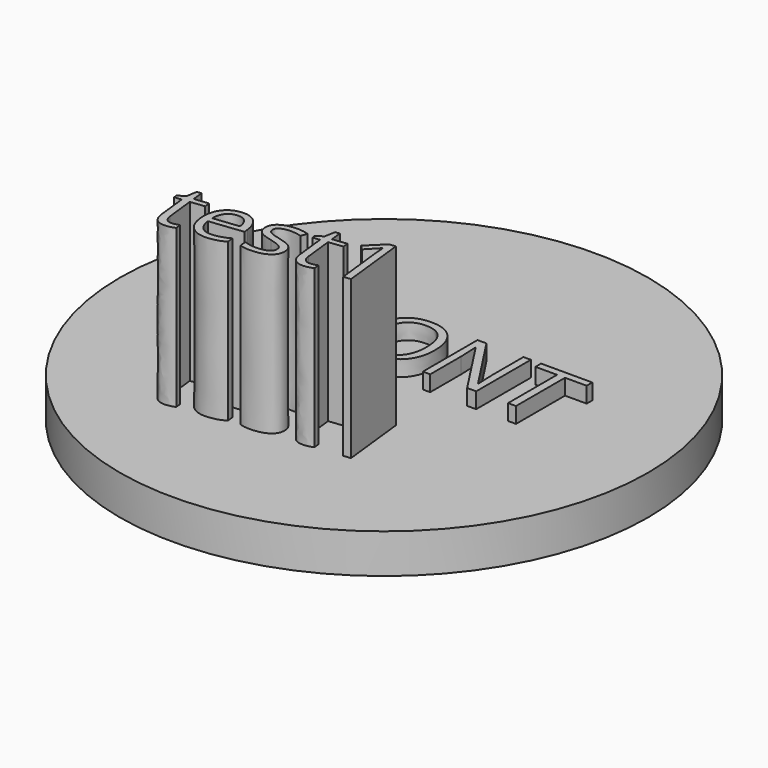
from build123d import *

# Parameters (mm, degrees)
F0_R         = 42.5666121287
F1_DEPTH     = 6.35
F2_TEXT_SIZE = 15.4234249041
F3_DEPTH     = 2.54
F4_TEXT_SIZE = 13.8114629937
F5_DEPTH     = 2.54
F6_TEXT_SIZE = 13.8114629937
F7_DEPTH     = 8.89
F8_TEXT_SIZE = 14.7895900429
F9_DEPTH     = 25.4


# Not quite as in the source:
# - Text() gives the source's letters only with a copy of the font that has no kerning and outlines rounded to 1/6400 em; it was checked with that copy


with BuildPart() as f1:
    # F0 (on Top) → F1 (new body)
    with BuildSketch(Plane.XY):
        Circle(F0_R)
    extrude(amount=F1_DEPTH)

    # F2 (on face) → F3 (join)
    with BuildSketch(Plane.XY.offset(6.35)):
        with Locations((-24.7606217465, 0)):
            Text('FRONT', F2_TEXT_SIZE, font='Open Sans', text_align=(TextAlign.LEFT, TextAlign.BOTTOM))
    extrude(amount=F3_DEPTH)

    # F4 (on face) → F5 (join)
    with BuildSketch(Plane(origin=(0, 0, 0), x_dir=(1, 0, 0), z_dir=(0, 0, -1))):
        with Locations(Location((-4.9150859907, 4.1357969787), (0, 0, 180))):
            Text('BACK', F4_TEXT_SIZE, font='Open Sans', text_align=(TextAlign.LEFT, TextAlign.BOTTOM))
        with Locations(Location((18.3764435351, -17.4402090912), (0, 0, 90))):
            Text('BACK', F4_TEXT_SIZE, font='Open Sans', text_align=(TextAlign.LEFT, TextAlign.BOTTOM))
        with Locations(Location((9.6465877128, 36.9843788118), (0, 0, -141.1464774033))):
            Text('BACK', F4_TEXT_SIZE, font='Open Sans', text_align=(TextAlign.LEFT, TextAlign.BOTTOM))
    extrude(amount=F5_DEPTH)

    # F6 (on face) → F7 (join, through all)
    with BuildSketch(Plane.XY.offset(6.35)):
        with Locations((-30.5778705515, 12.418014243)):
            Text('BACK', F6_TEXT_SIZE, font='Open Sans', text_align=(TextAlign.LEFT, TextAlign.BOTTOM))
    extrude(amount=-F7_DEPTH)

    # F8 (on face) → F9 (join)
    with BuildSketch(Plane.XY.offset(6.35)):
        with Locations(Location((-19.8778916181, -23.7059950025), (0, 0, 6.414713331))):
            Text('test1', F8_TEXT_SIZE, font='Open Sans', text_align=(TextAlign.LEFT, TextAlign.BOTTOM))
    extrude(amount=F9_DEPTH)


solid = f1.part
